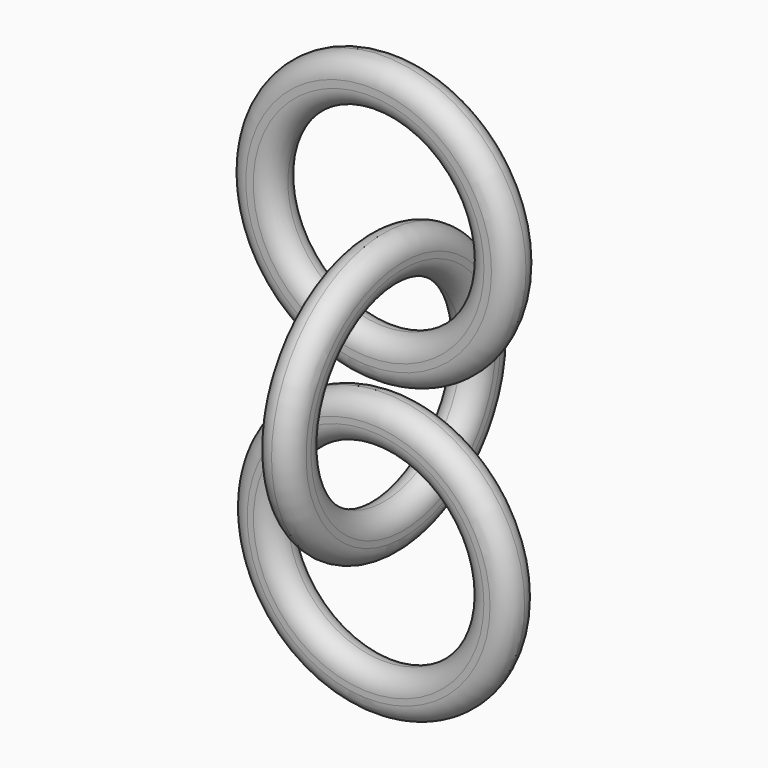
from build123d import *

# Parameters (mm, degrees)
F0_R     = 25.6374683223
F0_R_2   = 17.5110166509
F1_DEPTH = 3.5
F2_R     = 25.6372857839
F2_R_2   = 17.5089394863
F3_DEPTH = 3.5
F4_R     = 25.8993554988
F4_R_2   = 17.5369714652
F5_DEPTH = 3.5
F6_R     = 3.49999
F6_2_R   = 3.49999
F6_3_R   = 3.49999


# Not quite as in the source:
# - a fillet or chamfer is up to 0.001 mm smaller than in the source, because OpenCascade refuses the exact size


with BuildPart() as f1:
    # F0 (on Right) → F1 (new body, symmetric)
    with BuildSketch(Plane.YZ):
        Circle(F0_R)
        Circle(F0_R_2, mode=Mode.SUBTRACT)
    extrude(amount=F1_DEPTH, both=True)

    # F6#3 (radius 3.5 in the source; OpenCascade refuses exactly that, so slightly less here)
    f6_3_edges = [f1.edges().sort_by_distance(p)[0] for p in [
        (3.5, -25.637468, 0),
        (3.5, -17.511017, 0),
        (-3.5, -25.637468, 0),
        (-3.5, -17.511017, 0),
    ]]
    fillet(f6_3_edges, radius=F6_3_R)


with BuildPart() as f3:
    # F2 (on Front) → F3 (new body, symmetric)
    with BuildSketch(Plane.XZ):
        with Locations((0, -25.6372857839)):
            Circle(F2_R)
        with Locations((0, -25.6372857839)):
            Circle(F2_R_2, mode=Mode.SUBTRACT)
    extrude(amount=F3_DEPTH, both=True)

    # F6#2 (radius 3.5 in the source; OpenCascade refuses exactly that, so slightly less here)
    f6_2_edges = [f3.edges().sort_by_distance(p)[0] for p in [
        (-17.508939, -3.5, -25.637286),
        (17.508939, 0, -25.637286),
        (-17.508939, 3.5, -25.637286),
        (-25.637286, 3.5, -25.637286),
        (25.637286, 0, -25.637286),
        (-25.637286, -3.5, -25.637286),
    ]]
    fillet(f6_2_edges, radius=F6_2_R)


with BuildPart() as f5:
    # F4 (on Front) → F5 (new body, symmetric)
    with BuildSketch(Plane.XZ):
        with Locations((0, 28.152640909)):
            Circle(F4_R)
        with Locations((0, 28.152640909)):
            Circle(F4_R_2, mode=Mode.SUBTRACT)
    extrude(amount=F5_DEPTH, both=True)

    # F6 (radius 3.5 in the source; OpenCascade refuses exactly that, so slightly less here)
    f6_edges = [f5.edges().sort_by_distance(p)[0] for p in [
        (-25.899355, -3.5, 28.152641),
        (-25.899355, 3.5, 28.152641),
        (-17.536971, -3.5, 28.152641),
        (17.536971, 0, 28.152641),
        (-17.536971, 3.5, 28.152641),
    ]]
    fillet(f6_edges, radius=F6_R)


solid = Compound([f1.part, f3.part, f5.part])
